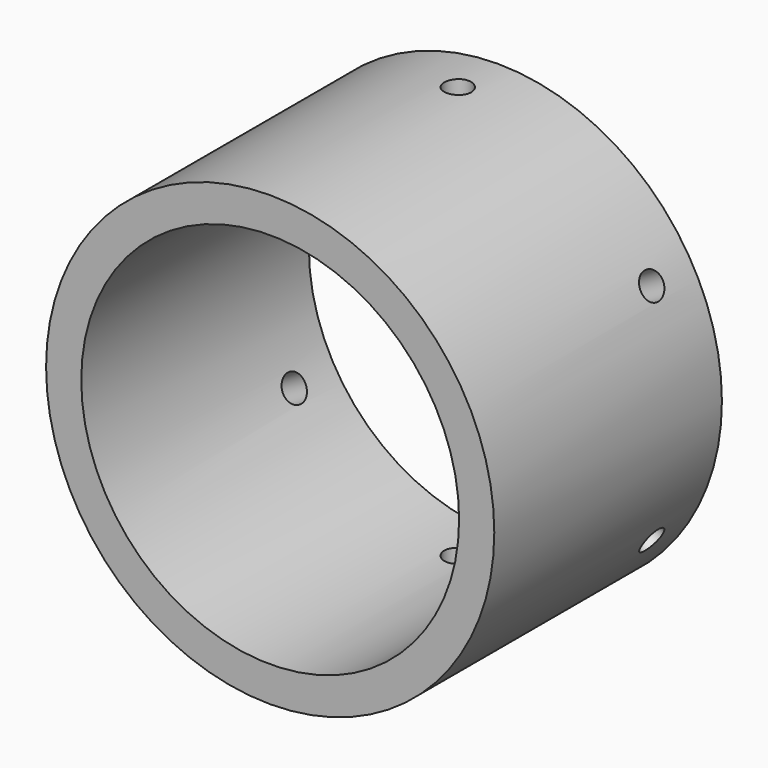
from build123d import *

# Parameters (mm, degrees)
F0_R            = 25.0063
F0_R_2          = 21.082
F1_DEPTH        = 31.75
F2_R            = 1.5
F3_DEPTH        = 25.4
F3_COPIES_COUNT = 6


# Not quite as in the source:
# - a pattern or mirror of a feature is missing from the dataset's text; its kind, count and spacing are read off the source's solid


with BuildPart() as f1:
    # F0 (on Front) → F1 (new body)
    with BuildSketch(Plane.XZ):
        Circle(F0_R)
        Circle(F0_R_2, mode=Mode.SUBTRACT)
    extrude(amount=F1_DEPTH)

    # F2 (on Top) → F3 (cut)
    with BuildSketch(Plane.XY):
        with Locations((0, -5.588)):
            Circle(F2_R)
    f3 = extrude(amount=F3_DEPTH, mode=Mode.SUBTRACT)

    # F3_copies: F3 ×6 about axis
    f3_copies_axis = Axis((0, 0, 0), (0, 1, 0))
    for i in range(1, F3_COPIES_COUNT):
        add(f3.rotate(f3_copies_axis, i * 360 / F3_COPIES_COUNT), mode=Mode.SUBTRACT)


solid = f1.part
